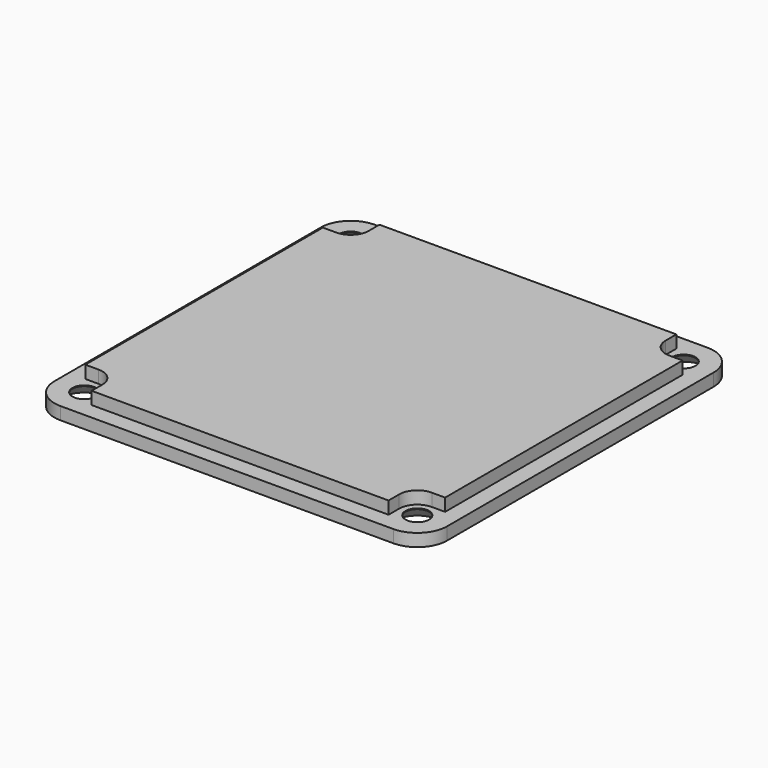
from build123d import *

# Parameters (mm, degrees)
F2_DEPTH                 = 1.6
F1_R                     = 1.5
F3_DEPTH                 = 1.6
F4_R                     = 3
F5_DEPTH                 = 25
DRAFT_F5_DRAFTED_ANGLE   = 45
DRAFT_F5_2_DRAFTED_ANGLE = 45
DRAFT_F5_3_DRAFTED_ANGLE = 45
DRAFT_F5_4_DRAFTED_ANGLE = 45


# Not quite as in the source:
# - an extrude with a draft is written as a straight extrude whose walls are then drafted


with BuildPart() as f2:
    # F1 (on Top) → F2 (new body)
    with BuildSketch(Plane.XY):
        with BuildLine():
            Line((18.9, 22.9), (0, 22.9))
            Line((0, 22.9), (-18.9, 22.9))
            Line((-18.9, 22.9), (-18.9, 21.2))
            ThreePointArc((-18.9, 21.2), (-19.5736544033, 19.5736544033), (-21.2, 18.9))
            Line((-21.2, 18.9), (-22.9, 18.9))
            Line((-22.9, 18.9), (-22.9, 0))
            Line((-22.9, 0), (-22.9, -18.9))
            Line((-22.9, -18.9), (-21.2, -18.9))
            ThreePointArc((-21.2, -18.9), (-19.5736544033, -19.5736544033), (-18.9, -21.2))
            Line((-18.9, -21.2), (-18.9, -22.9))
            Line((-18.9, -22.9), (0, -22.9))
            Line((0, -22.9), (18.9, -22.9))
            Line((18.9, -22.9), (18.9, -21.2))
            ThreePointArc((18.9, -21.2), (19.5736544033, -19.5736544033), (21.2, -18.9))
            Line((21.2, -18.9), (22.9, -18.9))
            Line((22.9, -18.9), (22.9, 0))
            Line((22.9, 0), (22.9, 18.9))
            Line((22.9, 18.9), (21.2, 18.9))
            ThreePointArc((21.2, 18.9), (19.5736544033, 19.5736544033), (18.9, 21.2))
            Line((18.9, 21.2), (18.9, 22.9))
        make_face()
    extrude(amount=F2_DEPTH)

    # F1 (on Top) → F3 (join)
    with BuildSketch(Plane.XY):
        with BuildLine():
            Line((0, 25), (-21.2, 25))
            ThreePointArc((-21.2, 25), (-23.8870057685, 23.8870057685), (-25, 21.2))
            Line((-25, 21.2), (-25, 0))
            Line((-25, 0), (-25, -21.2))
            ThreePointArc((-25, -21.2), (-23.8870057685, -23.8870057685), (-21.2, -25))
            Line((-21.2, -25), (0, -25))
            Line((0, -25), (21.2, -25))
            ThreePointArc((21.2, -25), (23.8870057685, -23.8870057685), (25, -21.2))
            Line((25, -21.2), (25, 0))
            Line((25, 0), (25, 21.2))
            ThreePointArc((25, 21.2), (23.8870057685, 23.8870057685), (21.2, 25))
            Line((21.2, 25), (0, 25))
        make_face()
        with Locations((-21.2, -21.2)):
            Circle(F1_R, mode=Mode.SUBTRACT)
        with Locations((21.2, -21.2)):
            Circle(F1_R, mode=Mode.SUBTRACT)
        with Locations((-21.2, 21.2)):
            Circle(F1_R, mode=Mode.SUBTRACT)
        with BuildLine():
            Line((-18.9, 22.9), (0, 22.9))
            Line((0, 22.9), (18.9, 22.9))
            Line((18.9, 22.9), (18.9, 21.2))
            ThreePointArc((18.9, 21.2), (19.5736544033, 19.5736544033), (21.2, 18.9))
            Line((21.2, 18.9), (22.9, 18.9))
            Line((22.9, 18.9), (22.9, 0))
            Line((22.9, 0), (22.9, -18.9))
            Line((22.9, -18.9), (21.2, -18.9))
            ThreePointArc((21.2, -18.9), (19.5736544033, -19.5736544033), (18.9, -21.2))
            Line((18.9, -21.2), (18.9, -22.9))
            Line((18.9, -22.9), (0, -22.9))
            Line((0, -22.9), (-18.9, -22.9))
            Line((-18.9, -22.9), (-18.9, -21.2))
            ThreePointArc((-18.9, -21.2), (-19.5736544033, -19.5736544033), (-21.2, -18.9))
            Line((-21.2, -18.9), (-22.9, -18.9))
            Line((-22.9, -18.9), (-22.9, 0))
            Line((-22.9, 0), (-22.9, 18.9))
            Line((-22.9, 18.9), (-21.2, 18.9))
            ThreePointArc((-21.2, 18.9), (-19.5736544033, 19.5736544033), (-18.9, 21.2))
            Line((-18.9, 21.2), (-18.9, 22.9))
        make_face(mode=Mode.SUBTRACT)
        with Locations((21.2, 21.2)):
            Circle(F1_R, mode=Mode.SUBTRACT)
        with BuildLine():
            Line((18.9, 22.9), (0, 22.9))
            Line((0, 22.9), (-18.9, 22.9))
            Line((-18.9, 22.9), (-18.9, 21.2))
            ThreePointArc((-18.9, 21.2), (-19.5736544033, 19.5736544033), (-21.2, 18.9))
            Line((-21.2, 18.9), (-22.9, 18.9))
            Line((-22.9, 18.9), (-22.9, 0))
            Line((-22.9, 0), (-22.9, -18.9))
            Line((-22.9, -18.9), (-21.2, -18.9))
            ThreePointArc((-21.2, -18.9), (-19.5736544033, -19.5736544033), (-18.9, -21.2))
            Line((-18.9, -21.2), (-18.9, -22.9))
            Line((-18.9, -22.9), (0, -22.9))
            Line((0, -22.9), (18.9, -22.9))
            Line((18.9, -22.9), (18.9, -21.2))
            ThreePointArc((18.9, -21.2), (19.5736544033, -19.5736544033), (21.2, -18.9))
            Line((21.2, -18.9), (22.9, -18.9))
            Line((22.9, -18.9), (22.9, 0))
            Line((22.9, 0), (22.9, 18.9))
            Line((22.9, 18.9), (21.2, 18.9))
            ThreePointArc((21.2, 18.9), (19.5736544033, 19.5736544033), (18.9, 21.2))
            Line((18.9, 21.2), (18.9, 22.9))
        make_face()
    extrude(amount=-F3_DEPTH)


with BuildPart() as f5_drafted:
    # F4 (on face) → F5 (new body)
    with BuildSketch(Plane(origin=(0, 0, -1.6), x_dir=(1, 0, 0), z_dir=(0, 0, -1))):
        with Locations((-21.2, 21.2)):
            Circle(F4_R)
    extrude(amount=-F5_DEPTH)

    # draft_F5_drafted
    draft_f5_drafted_walls = [f5_drafted.faces().sort_by_distance(p)[0] for p in [
        (-24.2, -21.2, 15.0666666667),
    ]]
    draft(draft_f5_drafted_walls, neutral_plane=Plane.XY.offset(-1.6), angle=DRAFT_F5_DRAFTED_ANGLE)


with BuildPart() as f2_1:
    add(f2.part)

    # join_F5_drafted: cut F5_drafted
    add(f5_drafted.part, mode=Mode.SUBTRACT)


with BuildPart() as f5_2_drafted:
    # F4 (on face) → F5, piece 2 (new body)
    with BuildSketch(Plane(origin=(0, 0, -1.6), x_dir=(1, 0, 0), z_dir=(0, 0, -1))):
        with Locations((21.2, 21.2)):
            Circle(F4_R)
    extrude(amount=-F5_DEPTH)

    # draft_F5_2_drafted
    draft_f5_2_drafted_walls = [f5_2_drafted.faces().sort_by_distance(p)[0] for p in [
        (18.2, -21.2, 15.0666666667),
    ]]
    draft(draft_f5_2_drafted_walls, neutral_plane=Plane.XY.offset(-1.6), angle=DRAFT_F5_2_DRAFTED_ANGLE)


with BuildPart() as f2_2:
    add(f2_1.part)

    # join_F5_2_drafted: cut F5_2_drafted
    add(f5_2_drafted.part, mode=Mode.SUBTRACT)


with BuildPart() as f5_3_drafted:
    # F4 (on face) → F5, piece 3 (new body)
    with BuildSketch(Plane(origin=(0, 0, -1.6), x_dir=(1, 0, 0), z_dir=(0, 0, -1))):
        with Locations((21.2, -21.2)):
            Circle(F4_R)
    extrude(amount=-F5_DEPTH)

    # draft_F5_3_drafted
    draft_f5_3_drafted_walls = [f5_3_drafted.faces().sort_by_distance(p)[0] for p in [
        (18.2, 21.2, 15.0666666667),
    ]]
    draft(draft_f5_3_drafted_walls, neutral_plane=Plane.XY.offset(-1.6), angle=DRAFT_F5_3_DRAFTED_ANGLE)


with BuildPart() as f2_3:
    add(f2_2.part)

    # join_F5_3_drafted: cut F5_3_drafted
    add(f5_3_drafted.part, mode=Mode.SUBTRACT)


with BuildPart() as f5_4_drafted:
    # F4 (on face) → F5, piece 4 (new body)
    with BuildSketch(Plane(origin=(0, 0, -1.6), x_dir=(1, 0, 0), z_dir=(0, 0, -1))):
        with Locations((-21.2, -21.2)):
            Circle(F4_R)
    extrude(amount=-F5_DEPTH)

    # draft_F5_4_drafted
    draft_f5_4_drafted_walls = [f5_4_drafted.faces().sort_by_distance(p)[0] for p in [
        (-24.2, 21.2, 15.0666666667),
    ]]
    draft(draft_f5_4_drafted_walls, neutral_plane=Plane.XY.offset(-1.6), angle=DRAFT_F5_4_DRAFTED_ANGLE)


with BuildPart() as f2_4:
    add(f2_3.part)

    # join_F5_4_drafted: cut F5_4_drafted
    add(f5_4_drafted.part, mode=Mode.SUBTRACT)


solid = f2_4.part
